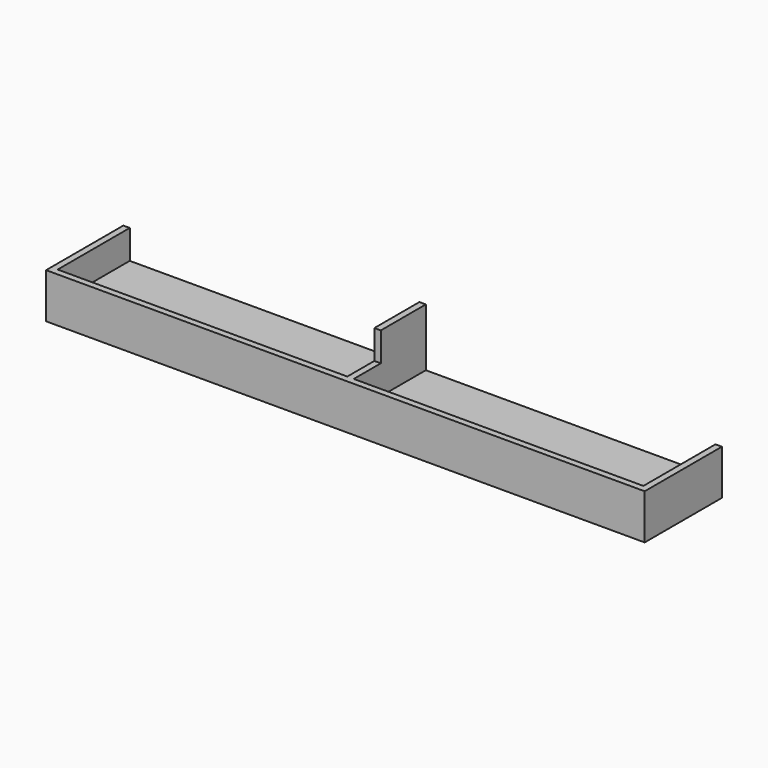
from build123d import *

# Parameters (mm, degrees)
F1_DEPTH = 500
F0_W     = 9000
F0_H     = 200
F0_W_2   = 200
F0_H_2   = 1050
F2_DEPTH = 1400
F0_H_3   = 1750
F3_DEPTH = 2300


with BuildPart() as f1:
    # F0 (on Top) → F1 (new body)
    with BuildSketch(Plane.XY):
        Polygon((-100, -250), (-100, 1500), (-9100, 1500), (-9100, -1300), (-100, -1300), align=None)
    extrude(amount=F1_DEPTH)



with BuildPart() as f1b:
    # F0 (on Top) → F1, piece 2 (new body)
    with BuildSketch(Plane.XY):
        Polygon((9100, -1300), (9100, 1500), (100, 1500), (100, -250), (100, -1300), align=None)
    extrude(amount=F1_DEPTH)


with BuildPart() as f2:
    # F0 (on Top) → F2 (new body)
    with BuildSketch(Plane.XY):
        Polygon((-9100, -1300), (-9100, 1500), (-9300, 1500), (-9300, -1500), (-9100, -1500), align=None)
        with Locations((-4600, -1400)):
            Rectangle(F0_W, F0_H)
        Polygon((9300, -1500), (9300, 1500), (9100, 1500), (9100, -1300), (9100, -1500), align=None)
        with Locations((4600, -1400)):
            Rectangle(F0_W, F0_H)
        with Locations((0, -1400)):
            Rectangle(F0_W_2, F0_H)
        with Locations((0, -775)):
            Rectangle(F0_W_2, F0_H_2)
    extrude(amount=F2_DEPTH)


with BuildPart() as f1_1:
    add(f1.part)

    add(f1b.part)  # F3 merges F1b

    add(f2.part)  # F3 merges F2
    # F0 (on Top) → F3 (join)
    with BuildSketch(Plane.XY):
        with Locations((0, 625)):
            Rectangle(F0_W_2, F0_H_3)
    extrude(amount=F3_DEPTH)


solid = f1_1.part
